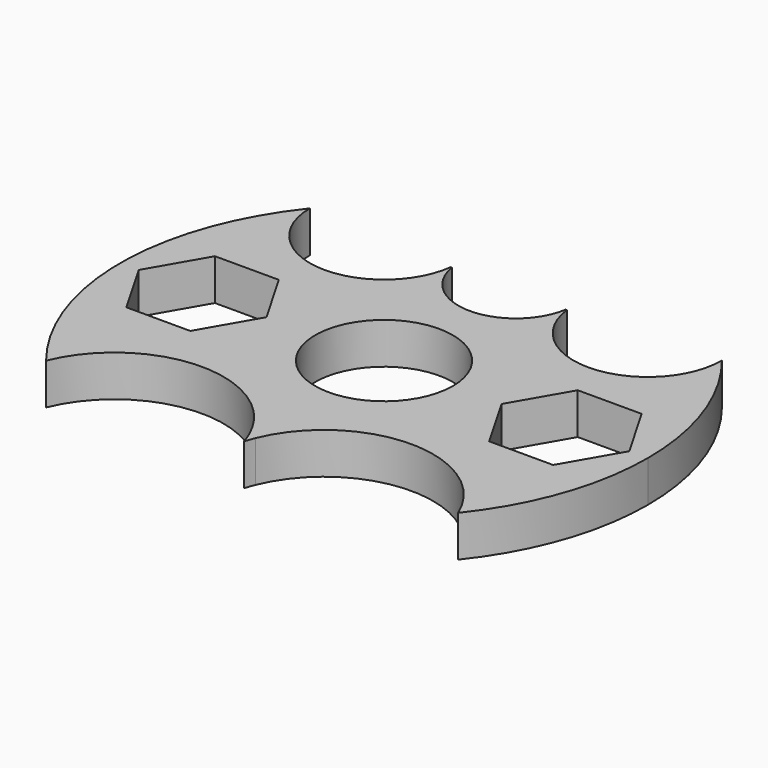
from build123d import *

# Parameters (mm, degrees)
F0_R     = 8.35
F1_DEPTH = 5


with BuildPart() as f1:
    # F0 (on Top) → F1 (new body)
    with BuildSketch(Plane.XY):
        with BuildLine():
            ThreePointArc((24.9799919936, -20), (30.1940370255, -10.5981190832), (32, 0))
            ThreePointArc((32, 0), (30.1940370255, 10.5981190832), (24.9799919936, 20))
            Line((24.9799919936, 20), (24.9799919936, 6.7116968793))
            Line((24.9799919936, 6.7116968793), (25.875, 6.7116968793))
            Line((25.875, 6.7116968793), (29.75, 0))
            Line((29.75, 0), (25.875, -6.7116968793))
            Line((25.875, -6.7116968793), (24.9799919936, -6.7116968793))
            Line((24.9799919936, -6.7116968793), (24.9799919936, -20))
        make_face()
        with BuildLine():
            Line((24.9799919936, 6.7116968793), (24.9799919936, 20))
            ThreePointArc((24.9799919936, 20), (16.5310257714, 11.0168846286), (7.0474671546, 18.9))
            Line((7.0474671546, 18.9), (6.8927707223, 18.9))
            ThreePointArc((6.8927707223, 18.9), (0, 13.0200080064), (-6.8927707223, 18.9))
            Line((-6.8927707223, 18.9), (-7.0474671546, 18.9))
            ThreePointArc((-7.0474671546, 18.9), (-16.5310257714, 11.0168846286), (-24.9799919936, 20))
            Line((-24.9799919936, 20), (-24.9799919936, 6.7116968793))
            Line((-24.9799919936, 6.7116968793), (-18.125, 6.7116968793))
            Line((-18.125, 6.7116968793), (-14.25, 0))
            Line((-14.25, 0), (-18.125, -6.7116968793))
            Line((-18.125, -6.7116968793), (-24.9799919936, -6.7116968793))
            Line((-24.9799919936, -6.7116968793), (-24.9799919936, -20))
            ThreePointArc((-24.9799919936, -20), (-12.7096008018, -11.75), (-0.43920961, -20))
            Line((-0.43920961, -20), (0.43920961, -20))
            ThreePointArc((0.43920961, -20), (12.7096008018, -11.75), (24.9799919936, -20))
            Line((24.9799919936, -20), (24.9799919936, -6.7116968793))
            Line((24.9799919936, -6.7116968793), (18.125, -6.7116968793))
            Line((18.125, -6.7116968793), (14.25, 0))
            Line((14.25, 0), (18.125, 6.7116968793))
            Line((18.125, 6.7116968793), (24.9799919936, 6.7116968793))
        make_face()
        Circle(F0_R, mode=Mode.SUBTRACT)
        with BuildLine():
            ThreePointArc((0, -21.2545297412), (0.2038636697, -20.6217539149), (0.43920961, -20))
            Line((0.43920961, -20), (-0.43920961, -20))
            ThreePointArc((-0.43920961, -20), (-0.2038636697, -20.6217539149), (0, -21.2545297412))
        make_face()
        with BuildLine():
            Line((-24.9799919936, 6.7116968793), (-24.9799919936, 20))
            ThreePointArc((-24.9799919936, 20), (-32, 0), (-24.9799919936, -20))
            Line((-24.9799919936, -20), (-24.9799919936, -6.7116968793))
            Line((-24.9799919936, -6.7116968793), (-25.875, -6.7116968793))
            Line((-25.875, -6.7116968793), (-29.75, 0))
            Line((-29.75, 0), (-25.875, 6.7116968793))
            Line((-25.875, 6.7116968793), (-24.9799919936, 6.7116968793))
        make_face()
    extrude(amount=F1_DEPTH)


solid = f1.part
